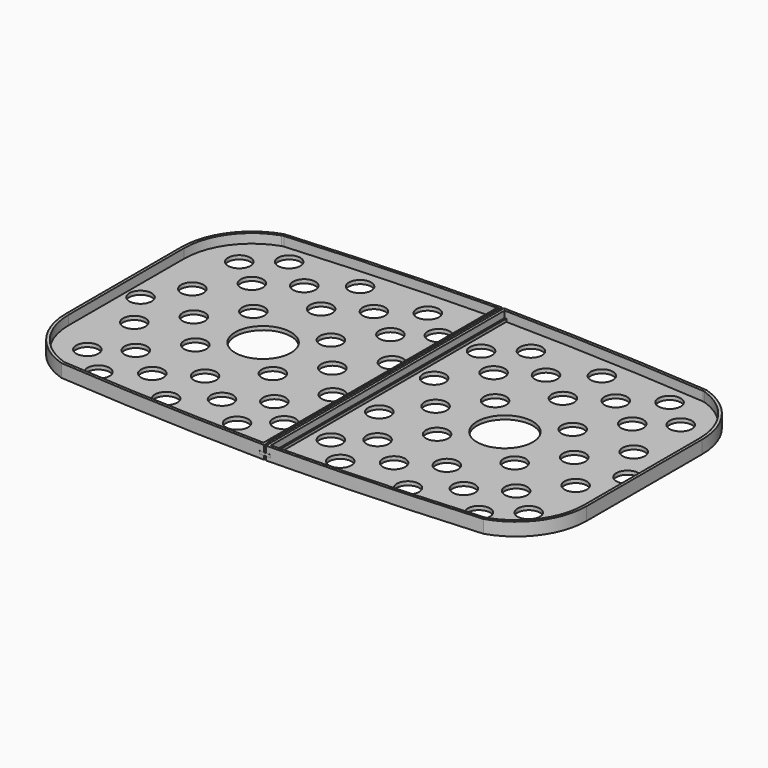
from build123d import *

# Parameters (mm, degrees)
F0_R     = 6
F0_R_2   = 15
F1_DEPTH = 2
F2_DEPTH = 5
F3_W     = 6
F3_H     = 160
F3_W_2   = 1
F3_H_2   = 154
F4_DEPTH = 1.5
F5_DEPTH = 6


with BuildPart() as f1:
    # F0 (on Top) → F1 (new body)
    with BuildSketch(Plane.XY):
        with BuildLine():
            Line((-0.5, 0), (-0.5, 79.9984374847))
            ThreePointArc((-0.5, 79.9984374847), (-57.0136629792, 78.37088801), (-113.4501771756, 75))
            ThreePointArc((-113.4501771756, 75), (-132.6521347762, 61.2260179571), (-140, 38.766128517))
            Line((-140, 38.766128517), (-140, 0))
            Line((-140, 0), (-140, -38.766128517))
            ThreePointArc((-140, -38.766128517), (-132.6521347762, -61.2260179571), (-113.4501771756, -75))
            ThreePointArc((-113.4501771756, -75), (-57.0136629792, -78.37088801), (-0.5, -79.9984374847))
            Line((-0.5, -79.9984374847), (-0.5, 0))
        make_face()
        with BuildLine():
            Line((-138.5, 0), (-138.5, 38.766128517))
            ThreePointArc((-138.5, 38.766128517), (-131.6867697088, 60.0016107168), (-113.790646342, 73.3092994606))
            ThreePointArc((-113.790646342, 73.3092994606), (-113.1776299217, 73.475900283), (-112.5484371493, 73.5634298262))
            ThreePointArc((-112.5484371493, 73.5634298262), (-57.311366893, 76.8562092122), (-2, 78.4776342095))
            Line((-2, 78.4776342095), (-2, 78.441327033))
            Line((-2, 78.441327033), (-2, 0.2514436209))
            Line((-2, 0.2514436209), (-2, -78.4413795778))
            Line((-2, -78.4413795778), (-2, -78.4776342095))
            ThreePointArc((-2, -78.4776342095), (-57.311366893, -76.8562092122), (-112.5484371493, -73.5634298262))
            ThreePointArc((-112.5484371493, -73.5634298262), (-113.1776299217, -73.475900283), (-113.790646342, -73.3092994606))
            ThreePointArc((-113.790646342, -73.3092994606), (-131.6867697088, -60.0016107168), (-138.5, -38.766128517))
            Line((-138.5, -38.766128517), (-138.5, 0))
        make_face(mode=Mode.SUBTRACT)
        with BuildLine():
            ThreePointArc((-113.790646342, 73.3092994606), (-131.6867697088, 60.0016107168), (-138.5, 38.766128517))
            Line((-138.5, 38.766128517), (-138.5, 0))
            Line((-138.5, 0), (-138.5, -38.766128517))
            ThreePointArc((-138.5, -38.766128517), (-131.6867697088, -60.0016107168), (-113.790646342, -73.3092994606))
            ThreePointArc((-113.790646342, -73.3092994606), (-113.1776299217, -73.475900283), (-112.5484371493, -73.5634298262))
            ThreePointArc((-112.5484371493, -73.5634298262), (-57.311366893, -76.8562092122), (-2, -78.4776342095))
            Line((-2, -78.4776342095), (-2, -78.4413795778))
            Line((-2, -78.4413795778), (-2, 0.2514436209))
            Line((-2, 0.2514436209), (-2, 78.441327033))
            Line((-2, 78.441327033), (-2, 78.4776342095))
            ThreePointArc((-2, 78.4776342095), (-57.311366893, 76.8562092122), (-112.5484371493, 73.5634298262))
            ThreePointArc((-112.5484371493, 73.5634298262), (-113.1776299217, 73.475900283), (-113.790646342, 73.3092994606))
        make_face()
        with Locations((-102.2574998881, -64.0849556577)):
            Circle(F0_R, mode=Mode.SUBTRACT)
        with Locations((-118.6551713943, -51.0527007282)):
            Circle(F0_R, mode=Mode.SUBTRACT)
        with Locations((-83.75, -51.0527007282)):
            Circle(F0_R, mode=Mode.SUBTRACT)
        with Locations((-65, -65.1682391763)):
            Circle(F0_R, mode=Mode.SUBTRACT)
        with Locations((-27.7425001119, -64.0849556577)):
            Circle(F0_R, mode=Mode.SUBTRACT)
        with Locations((-46.25, -51.0527007282)):
            Circle(F0_R, mode=Mode.SUBTRACT)
        with Locations((-12.4980853498, -51.3410195708)):
            Circle(F0_R, mode=Mode.SUBTRACT)
        with Locations((-102.2574998881, -39)):
            Circle(F0_R, mode=Mode.SUBTRACT)
        with Locations((-118.6551713943, -19.5)):
            Circle(F0_R, mode=Mode.SUBTRACT)
        with Locations((-85.8598283819, -19.5)):
            Circle(F0_R, mode=Mode.SUBTRACT)
        with Locations((-65, -39)):
            Circle(F0_R, mode=Mode.SUBTRACT)
        with Locations((-27.7425001119, -39)):
            Circle(F0_R, mode=Mode.SUBTRACT)
        with Locations((-44.1401716181, -19.5)):
            Circle(F0_R, mode=Mode.SUBTRACT)
        with Locations((-12.4980853498, -18.7883188426)):
            Circle(F0_R, mode=Mode.SUBTRACT)
        with Locations((-130.9094578028, 0)):
            Circle(F0_R, mode=Mode.SUBTRACT)
        with Locations((-118.6551713943, 19.5)):
            Circle(F0_R, mode=Mode.SUBTRACT)
        with Locations((-102.2574998881, 0)):
            Circle(F0_R, mode=Mode.SUBTRACT)
        with Locations((-85.8598283819, 19.5)):
            Circle(F0_R, mode=Mode.SUBTRACT)
        with Locations((-102.2574998881, 39)):
            Circle(F0_R, mode=Mode.SUBTRACT)
        with Locations((-65, 0)):
            Circle(F0_R_2, mode=Mode.SUBTRACT)
        with Locations((-44.1401716181, 19.5)):
            Circle(F0_R, mode=Mode.SUBTRACT)
        with Locations((-27.7425001119, 0)):
            Circle(F0_R, mode=Mode.SUBTRACT)
        with Locations((-11.3448286057, 19.5)):
            Circle(F0_R, mode=Mode.SUBTRACT)
        with Locations((-65, 39)):
            Circle(F0_R, mode=Mode.SUBTRACT)
        with Locations((-27.7425001119, 39)):
            Circle(F0_R, mode=Mode.SUBTRACT)
        with Locations((-118.6551713943, 51.0527007282)):
            Circle(F0_R, mode=Mode.SUBTRACT)
        with Locations((-83.75, 51.0527007282)):
            Circle(F0_R, mode=Mode.SUBTRACT)
        with Locations((-102.2574998881, 64.0849556577)):
            Circle(F0_R, mode=Mode.SUBTRACT)
        with Locations((-46.25, 51.0527007282)):
            Circle(F0_R, mode=Mode.SUBTRACT)
        with Locations((-11.3448286057, 51.0527007282)):
            Circle(F0_R, mode=Mode.SUBTRACT)
        with Locations((-65, 65.1682391763)):
            Circle(F0_R, mode=Mode.SUBTRACT)
        with Locations((-27.7425001119, 64.0849556577)):
            Circle(F0_R, mode=Mode.SUBTRACT)
    extrude(amount=-F1_DEPTH)

    # F0 (on Top) → F2, piece 2 (join)
    with BuildSketch(Plane.XY):
        with BuildLine():
            Line((-0.5, 0), (-0.5, 79.9984374847))
            ThreePointArc((-0.5, 79.9984374847), (-57.0136629792, 78.37088801), (-113.4501771756, 75))
            ThreePointArc((-113.4501771756, 75), (-132.6521347762, 61.2260179571), (-140, 38.766128517))
            Line((-140, 38.766128517), (-140, 0))
            Line((-140, 0), (-140, -38.766128517))
            ThreePointArc((-140, -38.766128517), (-132.6521347762, -61.2260179571), (-113.4501771756, -75))
            ThreePointArc((-113.4501771756, -75), (-57.0136629792, -78.37088801), (-0.5, -79.9984374847))
            Line((-0.5, -79.9984374847), (-0.5, 0))
        make_face()
        with BuildLine():
            Line((-138.5, 0), (-138.5, 38.766128517))
            ThreePointArc((-138.5, 38.766128517), (-131.6867697088, 60.0016107168), (-113.790646342, 73.3092994606))
            ThreePointArc((-113.790646342, 73.3092994606), (-113.1776299217, 73.475900283), (-112.5484371493, 73.5634298262))
            ThreePointArc((-112.5484371493, 73.5634298262), (-57.311366893, 76.8562092122), (-2, 78.4776342095))
            Line((-2, 78.4776342095), (-2, 78.441327033))
            Line((-2, 78.441327033), (-2, 0.2514436209))
            Line((-2, 0.2514436209), (-2, -78.4413795778))
            Line((-2, -78.4413795778), (-2, -78.4776342095))
            ThreePointArc((-2, -78.4776342095), (-57.311366893, -76.8562092122), (-112.5484371493, -73.5634298262))
            ThreePointArc((-112.5484371493, -73.5634298262), (-113.1776299217, -73.475900283), (-113.790646342, -73.3092994606))
            ThreePointArc((-113.790646342, -73.3092994606), (-131.6867697088, -60.0016107168), (-138.5, -38.766128517))
            Line((-138.5, -38.766128517), (-138.5, 0))
        make_face(mode=Mode.SUBTRACT)
    extrude(amount=F2_DEPTH)


with BuildPart() as f1b:
    # F0 (on Top) → F1, piece 2 (new body)
    with BuildSketch(Plane.XY):
        with BuildLine():
            Line((0.5, 79.9984374847), (0.5, 79.9917448723))
            Line((0.5, 79.9917448723), (0.5, 78.4983035398))
            Line((0.5, 78.4983035398), (0.5, 0))
            Line((0.5, 0), (0.5, -79.9984374847))
            ThreePointArc((0.5, -79.9984374847), (57.0136629792, -78.37088801), (113.4501771756, -75))
            ThreePointArc((113.4501771756, -75), (132.6521347762, -61.2260179571), (140, -38.766128517))
            Line((140, -38.766128517), (140, 0))
            Line((140, 0), (140, 38.766128517))
            ThreePointArc((140, 38.766128517), (132.6521347762, 61.2260179571), (113.4501771756, 75))
            ThreePointArc((113.4501771756, 75), (57.0136629792, 78.37088801), (0.5, 79.9984374847))
        make_face()
        with BuildLine():
            ThreePointArc((113.7766615915, 73.3140697257), (131.6824708211, 60.0076191887), (138.5, 38.766128517))
            Line((138.5, 38.766128517), (138.5, 0))
            Line((138.5, 0), (138.5, -38.766128517))
            ThreePointArc((138.5, -38.766128517), (131.6867697088, -60.0016107168), (113.790646342, -73.3092994606))
            ThreePointArc((113.790646342, -73.3092994606), (113.1776299217, -73.475900283), (112.5484371493, -73.5634298262))
            ThreePointArc((112.5484371493, -73.5634298262), (57.311366893, -76.8562092122), (2, -78.4776342095))
            Line((2, -78.4776342095), (2, -78.4413270176))
            Line((2, -78.4413270176), (2, 0.251443522))
            Line((2, 0.251443522), (2, 78.4776342095))
            ThreePointArc((2, 78.4776342095), (57.3177639293, 76.8559248338), (112.561208179, 73.5624745347))
            ThreePointArc((112.561208179, 73.5624745347), (113.1768279957, 73.4768933956), (113.7766615915, 73.3140697257))
        make_face(mode=Mode.SUBTRACT)
        with BuildLine():
            Line((138.5, 0), (138.5, 38.766128517))
            ThreePointArc((138.5, 38.766128517), (131.6824708211, 60.0076191887), (113.7766615915, 73.3140697257))
            ThreePointArc((113.7766615915, 73.3140697257), (113.1768279957, 73.4768933956), (112.561208179, 73.5624745347))
            ThreePointArc((112.561208179, 73.5624745347), (57.3177639293, 76.8559248338), (2, 78.4776342095))
            Line((2, 78.4776342095), (2, 0.251443522))
            Line((2, 0.251443522), (2, -78.4413270176))
            Line((2, -78.4413270176), (2, -78.4776342095))
            ThreePointArc((2, -78.4776342095), (57.311366893, -76.8562092122), (112.5484371493, -73.5634298262))
            ThreePointArc((112.5484371493, -73.5634298262), (113.1776299217, -73.475900283), (113.790646342, -73.3092994606))
            ThreePointArc((113.790646342, -73.3092994606), (131.6867697088, -60.0016107168), (138.5, -38.766128517))
            Line((138.5, -38.766128517), (138.5, 0))
        make_face()
        with Locations((27.7425001119, -64.0849556577)):
            Circle(F0_R, mode=Mode.SUBTRACT)
        with Locations((65, -65.1682391763)):
            Circle(F0_R, mode=Mode.SUBTRACT)
        with Locations((12.4980853498, -51.3410195708)):
            Circle(F0_R, mode=Mode.SUBTRACT)
        with Locations((46.25, -51.0527007282)):
            Circle(F0_R, mode=Mode.SUBTRACT)
        with Locations((102.2574998881, -64.0849556577)):
            Circle(F0_R, mode=Mode.SUBTRACT)
        with Locations((83.75, -51.0527007282)):
            Circle(F0_R, mode=Mode.SUBTRACT)
        with Locations((118.6551713943, -51.0527007282)):
            Circle(F0_R, mode=Mode.SUBTRACT)
        with Locations((27.7425001119, -39)):
            Circle(F0_R, mode=Mode.SUBTRACT)
        with Locations((65, -39)):
            Circle(F0_R, mode=Mode.SUBTRACT)
        with Locations((12.4980853498, -18.7883188426)):
            Circle(F0_R, mode=Mode.SUBTRACT)
        with Locations((44.1401716181, -19.5)):
            Circle(F0_R, mode=Mode.SUBTRACT)
        with Locations((102.2574998881, -39)):
            Circle(F0_R, mode=Mode.SUBTRACT)
        with Locations((85.8598283819, -19.5)):
            Circle(F0_R, mode=Mode.SUBTRACT)
        with Locations((118.6551713943, -19.5)):
            Circle(F0_R, mode=Mode.SUBTRACT)
        with Locations((27.7425001119, 0)):
            Circle(F0_R, mode=Mode.SUBTRACT)
        with Locations((11.3448286057, 19.5)):
            Circle(F0_R, mode=Mode.SUBTRACT)
        with Locations((65, 0)):
            Circle(F0_R_2, mode=Mode.SUBTRACT)
        with Locations((44.1401716181, 19.5)):
            Circle(F0_R, mode=Mode.SUBTRACT)
        with Locations((27.7425001119, 39)):
            Circle(F0_R, mode=Mode.SUBTRACT)
        with Locations((65, 39)):
            Circle(F0_R, mode=Mode.SUBTRACT)
        with Locations((102.2574998881, 0)):
            Circle(F0_R, mode=Mode.SUBTRACT)
        with Locations((85.8598283819, 19.5)):
            Circle(F0_R, mode=Mode.SUBTRACT)
        with Locations((130.9094578028, 0)):
            Circle(F0_R, mode=Mode.SUBTRACT)
        with Locations((118.6551713943, 19.5)):
            Circle(F0_R, mode=Mode.SUBTRACT)
        with Locations((102.2574998881, 39)):
            Circle(F0_R, mode=Mode.SUBTRACT)
        with Locations((11.3448286057, 51.0527007282)):
            Circle(F0_R, mode=Mode.SUBTRACT)
        with Locations((46.25, 51.0527007282)):
            Circle(F0_R, mode=Mode.SUBTRACT)
        with Locations((27.7425001119, 64.0849556577)):
            Circle(F0_R, mode=Mode.SUBTRACT)
        with Locations((65, 65.1682391763)):
            Circle(F0_R, mode=Mode.SUBTRACT)
        with Locations((83.75, 51.0527007282)):
            Circle(F0_R, mode=Mode.SUBTRACT)
        with Locations((118.6551713943, 51.0527007282)):
            Circle(F0_R, mode=Mode.SUBTRACT)
        with Locations((102.2574998881, 64.0849556577)):
            Circle(F0_R, mode=Mode.SUBTRACT)
    extrude(amount=-F1_DEPTH)

    # F0 (on Top) → F2 (join)
    with BuildSketch(Plane.XY):
        with BuildLine():
            Line((0.5, 79.9984374847), (0.5, 79.9917448723))
            Line((0.5, 79.9917448723), (0.5, 78.4983035398))
            Line((0.5, 78.4983035398), (0.5, 0))
            Line((0.5, 0), (0.5, -79.9984374847))
            ThreePointArc((0.5, -79.9984374847), (57.0136629792, -78.37088801), (113.4501771756, -75))
            ThreePointArc((113.4501771756, -75), (132.6521347762, -61.2260179571), (140, -38.766128517))
            Line((140, -38.766128517), (140, 0))
            Line((140, 0), (140, 38.766128517))
            ThreePointArc((140, 38.766128517), (132.6521347762, 61.2260179571), (113.4501771756, 75))
            ThreePointArc((113.4501771756, 75), (57.0136629792, 78.37088801), (0.5, 79.9984374847))
        make_face()
        with BuildLine():
            ThreePointArc((113.7766615915, 73.3140697257), (131.6824708211, 60.0076191887), (138.5, 38.766128517))
            Line((138.5, 38.766128517), (138.5, 0))
            Line((138.5, 0), (138.5, -38.766128517))
            ThreePointArc((138.5, -38.766128517), (131.6867697088, -60.0016107168), (113.790646342, -73.3092994606))
            ThreePointArc((113.790646342, -73.3092994606), (113.1776299217, -73.475900283), (112.5484371493, -73.5634298262))
            ThreePointArc((112.5484371493, -73.5634298262), (57.311366893, -76.8562092122), (2, -78.4776342095))
            Line((2, -78.4776342095), (2, -78.4413270176))
            Line((2, -78.4413270176), (2, 0.251443522))
            Line((2, 0.251443522), (2, 78.4776342095))
            ThreePointArc((2, 78.4776342095), (57.3177639293, 76.8559248338), (112.561208179, 73.5624745347))
            ThreePointArc((112.561208179, 73.5624745347), (113.1768279957, 73.4768933956), (113.7766615915, 73.3140697257))
        make_face(mode=Mode.SUBTRACT)
    extrude(amount=F2_DEPTH)


with BuildPart() as f4:
    # F3 (on Top) → F4 (new body)
    with BuildSketch(Plane.XY):
        Rectangle(F3_W, F3_H)
        Rectangle(F3_W_2, F3_H_2, mode=Mode.SUBTRACT)
        Rectangle(F3_W_2, F3_H_2)
    extrude(amount=F4_DEPTH)

    # F3 (on Top) → F5 (join)
    with BuildSketch(Plane.XY):
        Rectangle(F3_W_2, F3_H_2)
    extrude(amount=F5_DEPTH)


solid = Compound([f1.part, f1b.part, f4.part])
